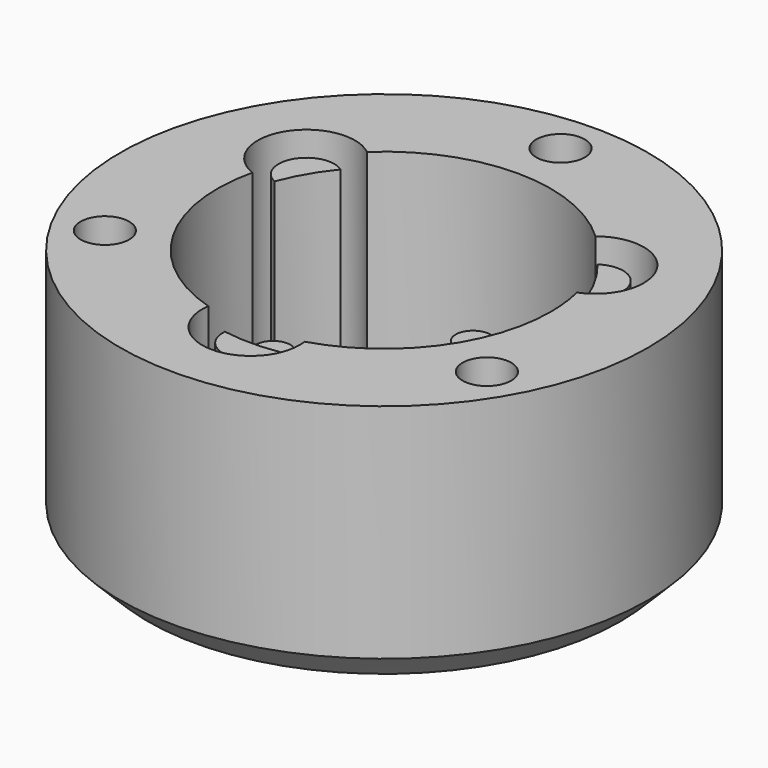
from build123d import *

# Parameters (mm, degrees)
F0_R         = 19
F0_R_2       = 1.75
F1_DEPTH     = 16
F0_R_3       = 1.25
F0_R_4       = 6
F1_FACE_R    = 19
F1_FACE_R_2  = 1.75
F1_FACE1_R   = 19
F1_FACE1_R_2 = 1.75
F2_DEPTH     = 2
F3_DEPTH     = 7
F5_DEPTH     = 15


# Not quite as in the source:
# - a fillet or chamfer that OpenCascade refuses, or shapes differently, is made with other operations: its cross-section is extruded or revolved along the edge and cut away or added


with BuildPart() as f1:
    # F0 (on Top) → F1 (new body)
    with BuildSketch(Plane.XY):
        Circle(F0_R)
        with Locations((-13.7481532851, -7.9375)):
            Circle(F0_R_2, mode=Mode.SUBTRACT)
        with BuildLine():
            ThreePointArc((11.6815620975, 2.746107602), (11.9201246883, 1.3822544682), (12, 0))
            ThreePointArc((12, 0), (9.6320035623, -7.1571298281), (3.4625821039, -11.4895833333))
            ThreePointArc((3.4625821039, -11.4895833333), (3.4906329916, -11.7441068228), (3.5, -12))
            ThreePointArc((3.5, -12), (-0.2558931772, -15.4906329916), (-3.4625821039, -11.4895833333))
            ThreePointArc((-3.4625821039, -11.4895833333), (-10.3923048454, -6), (-11.6815620975, 2.746107602))
            ThreePointArc((-11.6815620975, 2.746107602), (-13.4233937587, 7.75), (-8.2189799936, 8.7434757314))
            ThreePointArc((-8.2189799936, 8.7434757314), (0, 12), (8.2189799936, 8.7434757314))
            ThreePointArc((8.2189799936, 8.7434757314), (11.9160113491, 9.1509234346), (13.8923048454, 6))
            ThreePointArc((13.8923048454, 6), (13.2873351028, 4.0330735121), (11.6815620975, 2.746107602))
        make_face(mode=Mode.SUBTRACT)
        with Locations((13.7481532851, -7.9375)):
            Circle(F0_R_2, mode=Mode.SUBTRACT)
        with Locations((0, 15.875)):
            Circle(F0_R_2, mode=Mode.SUBTRACT)
    extrude(amount=F1_DEPTH)

    # F0 (on Top) + F1_face (on face) + F1_face1 (on face) → F2 (join)
    with BuildSketch(Plane.XY):
        Circle(F0_R)
        with Locations((-13.7481532851, -7.9375)):
            Circle(F0_R_2, mode=Mode.SUBTRACT)
        with BuildLine():
            ThreePointArc((11.6815620975, 2.746107602), (11.9201246883, 1.3822544682), (12, 0))
            ThreePointArc((12, 0), (9.6320035623, -7.1571298281), (3.4625821039, -11.4895833333))
            ThreePointArc((3.4625821039, -11.4895833333), (3.4906329916, -11.7441068228), (3.5, -12))
            ThreePointArc((3.5, -12), (-0.2558931772, -15.4906329916), (-3.4625821039, -11.4895833333))
            ThreePointArc((-3.4625821039, -11.4895833333), (-10.3923048454, -6), (-11.6815620975, 2.746107602))
            ThreePointArc((-11.6815620975, 2.746107602), (-13.4233937587, 7.75), (-8.2189799936, 8.7434757314))
            ThreePointArc((-8.2189799936, 8.7434757314), (0, 12), (8.2189799936, 8.7434757314))
            ThreePointArc((8.2189799936, 8.7434757314), (11.9160113491, 9.1509234346), (13.8923048454, 6))
            ThreePointArc((13.8923048454, 6), (13.2873351028, 4.0330735121), (11.6815620975, 2.746107602))
        make_face(mode=Mode.SUBTRACT)
        with Locations((13.7481532851, -7.9375)):
            Circle(F0_R_2, mode=Mode.SUBTRACT)
        with Locations((0, 15.875)):
            Circle(F0_R_2, mode=Mode.SUBTRACT)
        with BuildLine():
            ThreePointArc((3.4625821039, -11.4895833333), (9.6320035623, -7.1571298281), (12, 0))
            ThreePointArc((12, 0), (11.9201246883, 1.3822544682), (11.6815620975, 2.746107602))
            ThreePointArc((11.6815620975, 2.746107602), (7.3612159322, 4.25), (8.2189799936, 8.7434757314))
            ThreePointArc((8.2189799936, 8.7434757314), (0, 12), (-8.2189799936, 8.7434757314))
            ThreePointArc((-8.2189799936, 8.7434757314), (-7.2413814108, 7.5237065037), (-6.8923048454, 6))
            ThreePointArc((-6.8923048454, 6), (-8.4253783575, 3.1049697426), (-11.6815620975, 2.746107602))
            ThreePointArc((-11.6815620975, 2.746107602), (-10.3923048454, -6), (-3.4625821039, -11.4895833333))
            ThreePointArc((-3.4625821039, -11.4895833333), (-2.6659165155, -9.732206109), (-1.0590188837, -8.6640625))
            ThreePointArc((-1.0590188837, -8.6640625), (-0.3454897939, -6.79869371), (1.25, -8))
            ThreePointArc((1.25, -8), (1.20130629, -8.3454897939), (1.0590188837, -8.6640625))
            ThreePointArc((1.0590188837, -8.6640625), (2.6659165155, -9.732206109), (3.4625821039, -11.4895833333))
        make_face()
        with Locations((-8, 0)):
            Circle(F0_R_3, mode=Mode.SUBTRACT)
        Circle(F0_R_4, mode=Mode.SUBTRACT)
        with Locations((8, 0)):
            Circle(F0_R_3, mode=Mode.SUBTRACT)
        with Locations((0, 8)):
            Circle(F0_R_3, mode=Mode.SUBTRACT)
        with BuildLine():
            ThreePointArc((11.2444890067, 4.1906404019), (11.4857574222, 3.4752519965), (11.6815620975, 2.746107602))
            ThreePointArc((11.6815620975, 2.746107602), (13.2873351028, 4.0330735121), (13.8923048454, 6))
            ThreePointArc((13.8923048454, 6), (11.9160113491, 9.1509234346), (8.2189799936, 8.7434757314))
            ThreePointArc((8.2189799936, 8.7434757314), (8.7525352246, 8.2093317111), (9.2514455495, 7.6426929314))
            ThreePointArc((9.2514455495, 7.6426929314), (11.3192032779, 7.7722469624), (12.3923048454, 6))
            ThreePointArc((12.3923048454, 6), (12.0811459159, 4.928638325), (11.2444890067, 4.1906404019))
        make_face()
        with BuildLine():
            ThreePointArc((3.5, -12), (3.4906329916, -11.7441068228), (3.4625821039, -11.4895833333))
            ThreePointArc((3.4625821039, -11.4895833333), (2.7332221976, -11.6845837075), (1.9930434572, -11.8333333333))
            ThreePointArc((1.9930434572, -11.8333333333), (1.9982601075, -11.916594108), (2, -12))
            ThreePointArc((2, -12), (-0.083405892, -13.9982601075), (-1.9930434572, -11.8333333333))
            ThreePointArc((-1.9930434572, -11.8333333333), (-2.7332221976, -11.6845837075), (-3.4625821039, -11.4895833333))
            ThreePointArc((-3.4625821039, -11.4895833333), (-0.2558931772, -15.4906329916), (3.5, -12))
        make_face()
        with BuildLine():
            ThreePointArc((-9.2514455495, 7.6426929314), (-8.7525352246, 8.2093317111), (-8.2189799936, 8.7434757314))
            ThreePointArc((-8.2189799936, 8.7434757314), (-13.4233937587, 7.75), (-11.6815620975, 2.746107602))
            ThreePointArc((-11.6815620975, 2.746107602), (-11.4857574222, 3.4752519965), (-11.2444890067, 4.1906404019))
            ThreePointArc((-11.2444890067, 4.1906404019), (-12.124355653, 7), (-9.2514455495, 7.6426929314))
        make_face()
        with BuildLine():
            ThreePointArc((8.2189799936, 8.7434757314), (7.3612159322, 4.25), (11.6815620975, 2.746107602))
            ThreePointArc((11.6815620975, 2.746107602), (11.4857574222, 3.4752519965), (11.2444890067, 4.1906404019))
            ThreePointArc((11.2444890067, 4.1906404019), (8.6602540378, 5), (9.2514455495, 7.6426929314))
            ThreePointArc((9.2514455495, 7.6426929314), (8.7525352246, 8.2093317111), (8.2189799936, 8.7434757314))
        make_face()
        with BuildLine():
            ThreePointArc((-6.8923048454, 6), (-7.2413814108, 7.5237065037), (-8.2189799936, 8.7434757314))
            ThreePointArc((-8.2189799936, 8.7434757314), (-8.7525352246, 8.2093317111), (-9.2514455495, 7.6426929314))
            ThreePointArc((-9.2514455495, 7.6426929314), (-8.620057883, 6.9268984325), (-8.3923048454, 6))
            ThreePointArc((-8.3923048454, 6), (-9.3209431704, 4.3111589295), (-11.2444890067, 4.1906404019))
            ThreePointArc((-11.2444890067, 4.1906404019), (-11.4857574222, 3.4752519965), (-11.6815620975, 2.746107602))
            ThreePointArc((-11.6815620975, 2.746107602), (-8.4253783575, 3.1049697426), (-6.8923048454, 6))
        make_face()
        with BuildLine():
            ThreePointArc((1.9930434572, -11.8333333333), (2.7332221976, -11.6845837075), (3.4625821039, -11.4895833333))
            ThreePointArc((3.4625821039, -11.4895833333), (2.6659165155, -9.732206109), (1.0590188837, -8.6640625))
            ThreePointArc((1.0590188837, -8.6640625), (0, -9.25), (-1.0590188837, -8.6640625))
            ThreePointArc((-1.0590188837, -8.6640625), (-2.6659165155, -9.732206109), (-3.4625821039, -11.4895833333))
            ThreePointArc((-3.4625821039, -11.4895833333), (-2.7332221976, -11.6845837075), (-1.9930434572, -11.8333333333))
            ThreePointArc((-1.9930434572, -11.8333333333), (0, -10), (1.9930434572, -11.8333333333))
        make_face()
        with Locations((-13.7481532851, -7.9375)):
            Circle(F0_R_2)
        with Locations((13.7481532851, -7.9375)):
            Circle(F0_R_2)
        with Locations((0, 15.875)):
            Circle(F0_R_2)
        with BuildLine():
            ThreePointArc((9.2514455495, 7.6426929314), (10.3923048454, 6), (11.2444890067, 4.1906404019))
            ThreePointArc((11.2444890067, 4.1906404019), (12.0811459159, 4.928638325), (12.3923048454, 6))
            ThreePointArc((12.3923048454, 6), (11.3192032779, 7.7722469624), (9.2514455495, 7.6426929314))
        make_face()
        with BuildLine():
            ThreePointArc((-11.2444890067, 4.1906404019), (-10.3923048454, 6), (-9.2514455495, 7.6426929314))
            ThreePointArc((-9.2514455495, 7.6426929314), (-12.124355653, 7), (-11.2444890067, 4.1906404019))
        make_face()
        with BuildLine():
            ThreePointArc((2, -12), (1.9982601075, -11.916594108), (1.9930434572, -11.8333333333))
            ThreePointArc((1.9930434572, -11.8333333333), (0, -12), (-1.9930434572, -11.8333333333))
            ThreePointArc((-1.9930434572, -11.8333333333), (-0.083405892, -13.9982601075), (2, -12))
        make_face()
        with BuildLine():
            ThreePointArc((9.2514455495, 7.6426929314), (8.6602540378, 5), (11.2444890067, 4.1906404019))
            ThreePointArc((11.2444890067, 4.1906404019), (10.3923048454, 6), (9.2514455495, 7.6426929314))
        make_face()
        with BuildLine():
            ThreePointArc((-8.3923048454, 6), (-8.620057883, 6.9268984325), (-9.2514455495, 7.6426929314))
            ThreePointArc((-9.2514455495, 7.6426929314), (-10.3923048454, 6), (-11.2444890067, 4.1906404019))
            ThreePointArc((-11.2444890067, 4.1906404019), (-9.3209431704, 4.3111589295), (-8.3923048454, 6))
        make_face()
        with BuildLine():
            ThreePointArc((-1.9930434572, -11.8333333333), (0, -12), (1.9930434572, -11.8333333333))
            ThreePointArc((1.9930434572, -11.8333333333), (0, -10), (-1.9930434572, -11.8333333333))
        make_face()
        with Locations((0, 8)):
            Circle(F0_R_3)
        with Locations((8, 0)):
            Circle(F0_R_3)
        with Locations((-8, 0)):
            Circle(F0_R_3)
        with BuildLine():
            ThreePointArc((-1.0590188837, -8.6640625), (0, -8.5), (1.0590188837, -8.6640625))
            ThreePointArc((1.0590188837, -8.6640625), (1.20130629, -8.3454897939), (1.25, -8))
            ThreePointArc((1.25, -8), (-0.3454897939, -6.79869371), (-1.0590188837, -8.6640625))
        make_face()
        with BuildLine():
            ThreePointArc((-1.0590188837, -8.6640625), (0, -9.25), (1.0590188837, -8.6640625))
            ThreePointArc((1.0590188837, -8.6640625), (0, -8.5), (-1.0590188837, -8.6640625))
        make_face()
    with BuildSketch(Plane(origin=(0, 0, 0), x_dir=(1, 0, 0), z_dir=(0, 0, -1))):
        Circle(F1_FACE_R)
        with Locations((-13.7481532851, 7.9375)):
            Circle(F1_FACE_R_2, mode=Mode.SUBTRACT)
        with BuildLine():
            ThreePointArc((-8.2189799936, -8.7434757314), (-13.4233937587, -7.75), (-11.6815620975, -2.746107602))
            ThreePointArc((-11.6815620975, -2.746107602), (-10.3923048454, 6), (-3.4625821039, 11.4895833333))
            ThreePointArc((-3.4625821039, 11.4895833333), (0, 15.5), (3.4625821039, 11.4895833333))
            ThreePointArc((3.4625821039, 11.4895833333), (10.3923048454, 6), (11.6815620975, -2.746107602))
            ThreePointArc((11.6815620975, -2.746107602), (13.4233937587, -7.75), (8.2189799936, -8.7434757314))
            ThreePointArc((8.2189799936, -8.7434757314), (0, -12), (-8.2189799936, -8.7434757314))
        make_face(mode=Mode.SUBTRACT)
        with Locations((13.7481532851, 7.9375)):
            Circle(F1_FACE_R_2, mode=Mode.SUBTRACT)
        with Locations((0, -15.875)):
            Circle(F1_FACE_R_2, mode=Mode.SUBTRACT)
    with BuildSketch(Plane.XY.offset(16)):
        Circle(F1_FACE1_R)
        with Locations((-13.7481532851, -7.9375)):
            Circle(F1_FACE1_R_2, mode=Mode.SUBTRACT)
        with BuildLine():
            ThreePointArc((-11.6815620975, 2.746107602), (-13.4233937587, 7.75), (-8.2189799936, 8.7434757314))
            ThreePointArc((-8.2189799936, 8.7434757314), (0, 12), (8.2189799936, 8.7434757314))
            ThreePointArc((8.2189799936, 8.7434757314), (13.4233937587, 7.75), (11.6815620975, 2.746107602))
            ThreePointArc((11.6815620975, 2.746107602), (10.3923048454, -6), (3.4625821039, -11.4895833333))
            ThreePointArc((3.4625821039, -11.4895833333), (0, -15.5), (-3.4625821039, -11.4895833333))
            ThreePointArc((-3.4625821039, -11.4895833333), (-10.3923048454, -6), (-11.6815620975, 2.746107602))
        make_face(mode=Mode.SUBTRACT)
        with Locations((13.7481532851, -7.9375)):
            Circle(F1_FACE1_R_2, mode=Mode.SUBTRACT)
        with Locations((0, 15.875)):
            Circle(F1_FACE1_R_2, mode=Mode.SUBTRACT)
    extrude(amount=-F2_DEPTH, dir=(0, 0, 1))

    # F0 (on Top) → F3 (join)
    with BuildSketch(Plane.XY):
        with Locations((-8, 0)):
            Circle(F0_R_3)
        with Locations((0, 8)):
            Circle(F0_R_3)
        with Locations((8, 0)):
            Circle(F0_R_3)
        with BuildLine():
            ThreePointArc((-1.0590188837, -8.6640625), (0, -8.5), (1.0590188837, -8.6640625))
            ThreePointArc((1.0590188837, -8.6640625), (1.20130629, -8.3454897939), (1.25, -8))
            ThreePointArc((1.25, -8), (-0.3454897939, -6.79869371), (-1.0590188837, -8.6640625))
        make_face()
        with BuildLine():
            ThreePointArc((-1.0590188837, -8.6640625), (0, -9.25), (1.0590188837, -8.6640625))
            ThreePointArc((1.0590188837, -8.6640625), (0, -8.5), (-1.0590188837, -8.6640625))
        make_face()
    extrude(amount=F3_DEPTH)

    # F4: chamfer of 2 on 1 edges, made by hand

    # F4_s1 → F4_t2 (revolve, cut)
    with BuildSketch(Plane.XZ):
        Polygon((19, 0), (17, -2), (19, -2), align=None)
    revolve(axis=Axis((0, 0, -2), (0, 0, 1)), mode=Mode.SUBTRACT)

    # F0 (on Top) → F5 (join)
    with BuildSketch(Plane.XY):
        with BuildLine():
            ThreePointArc((-11.2444890067, 4.1906404019), (-10.3923048454, 6), (-9.2514455495, 7.6426929314))
            ThreePointArc((-9.2514455495, 7.6426929314), (-12.124355653, 7), (-11.2444890067, 4.1906404019))
        make_face()
        with BuildLine():
            ThreePointArc((9.2514455495, 7.6426929314), (10.3923048454, 6), (11.2444890067, 4.1906404019))
            ThreePointArc((11.2444890067, 4.1906404019), (12.0811459159, 4.928638325), (12.3923048454, 6))
            ThreePointArc((12.3923048454, 6), (11.3192032779, 7.7722469624), (9.2514455495, 7.6426929314))
        make_face()
        with BuildLine():
            ThreePointArc((2, -12), (1.9982601075, -11.916594108), (1.9930434572, -11.8333333333))
            ThreePointArc((1.9930434572, -11.8333333333), (0, -12), (-1.9930434572, -11.8333333333))
            ThreePointArc((-1.9930434572, -11.8333333333), (-0.083405892, -13.9982601075), (2, -12))
        make_face()
    extrude(amount=F5_DEPTH)


solid = f1.part
